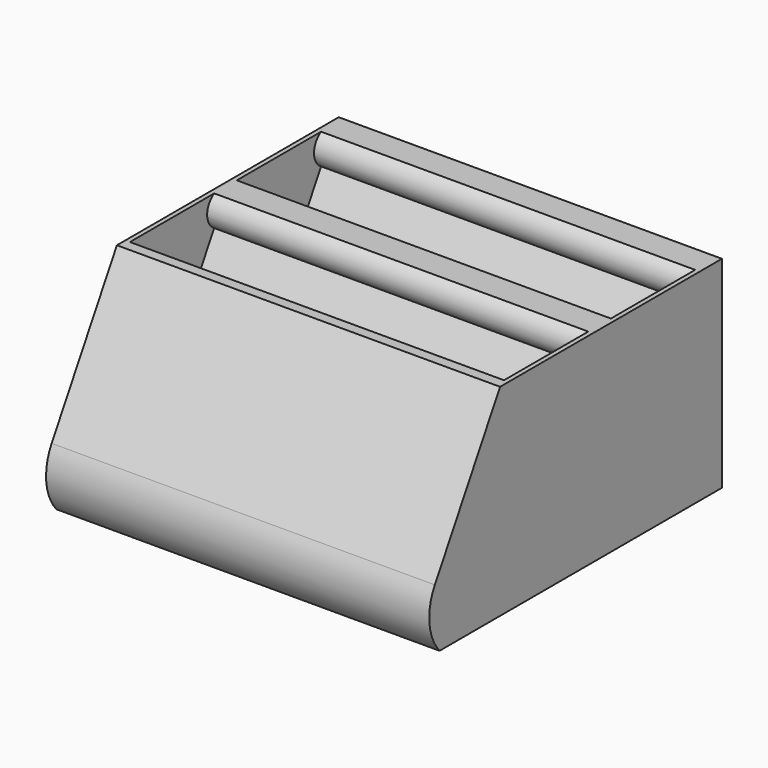
from build123d import *

# Parameters (mm, degrees)
F1_DEPTH     = 38
F4_DEPTH     = 74.2
F5_DEPTH     = 1
F6_DEPTH     = 1
F7_TEXT_SIZE = 14.9691813729
F8_DEPTH     = 0.5
F10_R        = 1
F12_DEPTH    = 74.2


# Not quite as in the source:
# - Text() gives the source's letters only with a copy of the font that has no kerning and outlines rounded to 1/6400 em; it was checked with that copy


with BuildPart() as f1:
    # F0 (on Right) → F1 (new body, symmetric)
    with BuildSketch(Plane.YZ):
        with BuildLine():
            ThreePointArc((-36.1727135145, 11.9880384966), (-37.5100817827, 5.8058334716), (-35, 0))
            Line((-35, 0), (35, 0))
            Line((35, 0), (35, 40))
            Line((35, 40), (-20, 40))
            Line((-20, 40), (-36.1727135145, 11.9880384966))
        make_face()
    extrude(amount=F1_DEPTH, both=True)

    # F3 (on offset) → F4 (cut)
    with BuildSketch(Plane.YZ.offset(37.1)):
        Polygon((6.5, 40), (-17.9, 40), (-34.0727135145, 11.9880384966), (-15.7727135145, 1.4225285704), align=None)
        Polygon((35, 40), (12.5678780843, 1.1464251204), (35, 1.1464251204), align=None)
        Polygon((33, 40), (8.6, 40), (-1.4727135145, 22.5535484227), (16.8272864855, 11.9880384966), align=None)
    extrude(amount=-F4_DEPTH, mode=Mode.SUBTRACT)

    # F5 (add): a face of the model
    f5_faces = [f1.faces().sort_by_distance(p)[0] for p in [
        (37.1, 27.5226260281, 14.0976167469),
    ]]
    extrude(f5_faces, amount=F5_DEPTH)

    # F6 (add): a face of the model
    f6_faces = [f1.faces().sort_by_distance(p)[0] for p in [
        (-37.1, 27.5226260281, 14.0976167469),
    ]]
    extrude(f6_faces, amount=F6_DEPTH)

    # F7 (on face) → F8 (join)
    with BuildSketch(Plane.XY.offset(1.1464251204)):
        with Locations((-13.2593465969, 20.5335263163)):
            Text('3E8', F7_TEXT_SIZE, font='Open Sans', text_align=(TextAlign.LEFT, TextAlign.BOTTOM))
    extrude(amount=F8_DEPTH)

    # F10
    f10_edges = [f1.edges().sort_by_distance(p)[0] for p in [
        (0, 12.567878, 1.146425),
    ]]
    fillet(f10_edges, radius=F10_R)

    # F11 (on face) → F12 (join, through all)
    with BuildSketch(Plane.YZ.offset(-37.1)):
        with BuildLine():
            Line((3, 33.9378221735), (6.5, 40))
            Line((6.5, 40), (3, 40))
            ThreePointArc((3, 40), (1.25, 36.9689110868), (3, 33.9378221735))
        make_face()
        with BuildLine():
            Line((29.5, 33.9378221735), (33, 40))
            Line((33, 40), (29.5, 40))
            ThreePointArc((29.5, 40), (27.75, 36.9689110868), (29.5, 33.9378221735))
        make_face()
        Polygon((-1.4727135145, 22.5535484227), (3.8369054287, 19.4880384966), (2.4773053326, 29.3951817568), align=None)
        Polygon((-34.0727135145, 11.9880384966), (-28.7630945713, 8.9225285704), (-30.1226946674, 18.8296718306), align=None)
    extrude(amount=F12_DEPTH)


solid = f1.part
